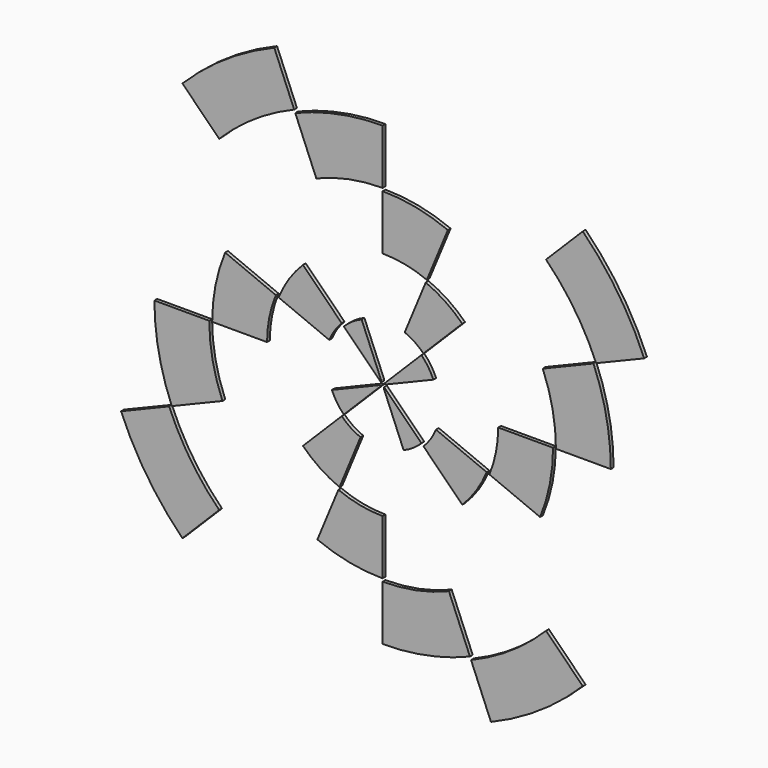
from build123d import *

# Parameters (mm, degrees)
F1_DEPTH = 1.2


# Not quite as in the source:
# - ends of sketch curves that miss each other by under 0.0002 mm in the source are joined


with BuildPart() as f1:
    # F0 (on Front) → F1 (new body)
    with BuildSketch(Plane.XZ):
        with BuildLine():
            Line((-1.2989994546, 0.0015044786), (15.0476048994, 6.7724896142))
            ThreePointArc((15.0476048994, 6.7724896142), (13.2918164287, 10.0573388369), (10.928922648, 12.9365332644))
            Line((10.928922648, 12.9365332644), (-2.0061062491, 0.0015044765))
            Line((-2.0061062498, 0.0015044786), (-1.2989994546, 0.0015044786))
        make_face()
    extrude(amount=F1_DEPTH)


with BuildPart() as f1b:
    # F0 (on Front) → F1, piece 2 (new body)
    with BuildSketch(Plane.XZ):
        with BuildLine():
            Line((11.6360294322, 13.6436400426), (25.0710583314, 27.0786688285))
            ThreePointArc((25.0710583314, 27.0786688285), (19.1611329685, 31.9288192702), (12.4185477522, 35.532806188))
            Line((12.4185477522, 35.532806188), (5.1475624685, 17.9790950988))
            ThreePointArc((5.1475624685, 17.9790950988), (8.6052984769, 16.1308966794), (11.6360294322, 13.6436400426))
        make_face()
    extrude(amount=F1_DEPTH)


with BuildPart() as f1c:
    # F0 (on Front) → F1, piece 3 (new body)
    with BuildSketch(Plane.XZ):
        with BuildLine():
            Line((12.8012311882, 36.4566857191), (20.0722164719, 54.0103968083))
            ThreePointArc((20.0722164719, 54.0103968083), (9.0042229134, 57.3678359894), (-2.5061061445, 58.5015044786))
            Line((-2.5061061445, 58.5015044786), (-2.5061062512, 39.5015044786))
            ThreePointArc((-2.5061062512, 39.5015044786), (5.2975067418, 38.7329156724), (12.8012311882, 36.4566857191))
        make_face()
    extrude(amount=F1_DEPTH)


with BuildPart() as f1d:
    # F0 (on Front) → F1, piece 4 (new body)
    with BuildSketch(Plane.XZ):
        with BuildLine():
            Line((-2.5061062512, 59.5015044786), (-2.5061062512, 78.5015044786))
            ThreePointArc((-2.5061062512, 78.5015044786), (-17.918241492, 76.9835416699), (-32.7380971661, 72.4879876471))
            Line((-32.7380971661, 72.4879876471), (-25.4671120094, 54.9342765053))
            ThreePointArc((-25.4671120094, 54.9342765053), (-14.2115254214, 58.3486213327), (-2.5061062512, 59.5015044786))
        make_face()
    extrude(amount=F1_DEPTH)


with BuildPart() as f1e:
    # F0 (on Front) → F1, piece 5 (new body)
    with BuildSketch(Plane.XZ):
        with BuildLine():
            ThreePointArc((-59.0746485757, 56.0700471439), (-46.9517246823, 66.0190736034), (-33.1207805954, 73.4118671809))
            Line((-33.1207805954, 73.4118671809), (-40.0090823229, 90.041698789))
            ThreePointArc((-40.0090823229, 90.041698789), (-56.9519888293, 80.9855266564), (-71.8025705987, 68.7979692436))
            Line((-71.8025705987, 68.7979692436), (-59.0746485757, 56.0700471439))
        make_face()
    extrude(amount=F1_DEPTH)


with BuildPart() as f1f:
    # F0 (on Front) → F1, piece 6 (new body)
    with BuildSketch(Plane.XZ):
        with BuildLine():
            Line((-15.9411350532, 12.9365333616), (-3.0061062497, 0.0015044801))
            Line((-3.0061062512, 0.0015044796), (-3.0061062512, 0.7086112711))
            Line((-3.0061062512, 0.7086112711), (-9.7770914079, 17.0552156204))
            ThreePointArc((-9.7770914079, 17.0552156204), (-13.0619406286, 15.2994271457), (-15.9411350532, 12.9365333616))
        make_face()
    extrude(amount=F1_DEPTH)


with BuildPart() as f1g:
    # F0 (on Front) → F1, piece 7 (new body)
    with BuildSketch(Plane.XZ):
        with BuildLine():
            Line((-16.6482418323, 13.6436401449), (-30.0832706344, 27.0786690279))
            ThreePointArc((-30.0832706344, 27.0786690279), (-34.933421069, 21.1687436591), (-38.5374079786, 14.4261584385))
            Line((-38.5374079786, 14.4261584385), (-20.9836968806, 7.155173176))
            ThreePointArc((-20.9836968806, 7.155173176), (-19.1354984654, 10.6129091865), (-16.6482418323, 13.6436401449))
        make_face()
    extrude(amount=F1_DEPTH)


with BuildPart() as f1h:
    # F0 (on Front) → F1, piece 8 (new body)
    with BuildSketch(Plane.XZ):
        with BuildLine():
            Line((-39.4612875101, 14.8088418734), (-57.0149986081, 22.0798271359))
            ThreePointArc((-57.0149986081, 22.0798271359), (-60.3724377655, 11.0118336257), (-61.5061062512, -0.4984953792))
            Line((-61.5061062512, -0.4984953792), (-42.5061062512, -0.498495425))
            ThreePointArc((-42.5061062512, -0.498495425), (-41.7375174473, 7.3051174597), (-39.4612875101, 14.8088418734))
        make_face()
    extrude(amount=F1_DEPTH)


with BuildPart() as f1i:
    # F0 (on Front) → F1, piece 9 (new body)
    with BuildSketch(Plane.XZ):
        with BuildLine():
            ThreePointArc((-81.5061062512, -0.498495331), (-79.9881434379, -15.9106307856), (-75.4925893833, -30.7304865244))
            Line((-75.4925893833, -30.7304865244), (-57.9388782503, -23.4595013464))
            ThreePointArc((-57.9388782503, -23.4595013464), (-61.3532231018, -12.2039147094), (-62.5061062512, -0.4984953768))
            Line((-62.5061062512, -0.4984953768), (-81.5061062512, -0.498495331))
        make_face()
    extrude(amount=F1_DEPTH)


with BuildPart() as f1j:
    # F0 (on Front) → F1, piece 10 (new body)
    with BuildSketch(Plane.XZ):
        with BuildLine():
            Line((-71.8025709327, -69.7949599525), (-59.0746488484, -57.0670379141))
            ThreePointArc((-59.0746488484, -57.0670379141), (-69.0236753224, -44.9441140327), (-76.4164689166, -31.1131699548))
            Line((-76.4164689166, -31.1131699548), (-93.0463005164, -38.0014717023))
            ThreePointArc((-93.0463005164, -38.0014717023), (-83.9901283634, -54.9443781978), (-71.8025709327, -69.7949599525))
        make_face()
    extrude(amount=F1_DEPTH)


with BuildPart() as f1k:
    # F0 (on Front) → F1, piece 11 (new body)
    with BuildSketch(Plane.XZ):
        with BuildLine():
            Line((-15.941135118, -13.9335243397), (-3.0061062521, -0.9984955205))
            Line((-3.0061062518, -0.9984955214), (-3.7132130396, -0.9984955214))
            Line((-3.7132130396, -0.9984955214), (-20.0598173842, -7.7694806994))
            ThreePointArc((-20.0598173842, -7.7694806994), (-18.3040289056, -11.0543299179), (-15.941135118, -13.9335243397))
        make_face()
    extrude(amount=F1_DEPTH)


with BuildPart() as f1l:
    # F0 (on Front) → F1, piece 12 (new body)
    with BuildSketch(Plane.XZ):
        with BuildLine():
            ThreePointArc((-30.0832707673, -28.0756599379), (-24.1733453927, -32.9258103653), (-17.4307601677, -36.5297972669))
            Line((-17.4307601677, -36.5297972669), (-10.1597749263, -18.9760861601))
            ThreePointArc((-10.1597749263, -18.9760861601), (-13.6175109391, -17.1278877491), (-16.6482419005, -14.6406311196))
            Line((-16.6482419005, -14.6406311196), (-30.0832707673, -28.0756599379))
        make_face()
    extrude(amount=F1_DEPTH)


with BuildPart() as f1m:
    # F0 (on Front) → F1, piece 13 (new body)
    with BuildSketch(Plane.XZ):
        with BuildLine():
            ThreePointArc((-25.0844288428, -55.0073879056), (-14.0164353111, -58.3648270531), (-2.5061062867, -59.4984955214))
            Line((-2.5061062512, -59.4984955214), (-2.5061062512, -40.4984955214))
            ThreePointArc((-2.5061062753, -40.4984955214), (-10.3097191732, -39.7299067293), (-17.8134436014, -37.4536767988))
            Line((-17.8134436014, -37.4536767988), (-25.0844288428, -55.0073879056))
        make_face()
    extrude(amount=F1_DEPTH)


with BuildPart() as f1n:
    # F0 (on Front) → F1, piece 14 (new body)
    with BuildSketch(Plane.XZ):
        with BuildLine():
            ThreePointArc((-2.5061062988, -79.4984955214), (12.9060291297, -77.9805326849), (27.7258848397, -73.4849786172))
            Line((27.7258848397, -73.4849786172), (20.4548996406, -55.9312674929))
            ThreePointArc((20.4548996406, -55.9312674929), (9.1993130255, -59.3456123544), (-2.5061062873, -60.4984955214))
            Line((-2.5061062512, -60.4984955214), (-2.5061062512, -79.4984955214))
        make_face()
    extrude(amount=F1_DEPTH)


with BuildPart() as f1o:
    # F0 (on Front) → F1, piece 15 (new body)
    with BuildSketch(Plane.XZ):
        with BuildLine():
            Line((66.7903582634, -69.7949601195), (54.0624362097, -57.0670380504))
            ThreePointArc((54.0624362097, -57.0670380504), (41.9395123403, -67.0160645391), (28.1085682712, -74.40885815))
            Line((28.1085682712, -74.40885815), (34.9968700388, -91.0386897414))
            ThreePointArc((34.9968700388, -91.0386897414), (51.9397765234, -81.9825175681), (66.7903582634, -69.7949601195))
        make_face()
    extrude(amount=F1_DEPTH)


with BuildPart() as f1p:
    # F0 (on Front) → F1, piece 16 (new body)
    with BuildSketch(Plane.XZ):
        with BuildLine():
            ThreePointArc((4.7648789479, -18.0522066457), (8.0497281643, -16.2964181631), (10.9289225833, -13.9335243721))
            Line((10.9289225833, -13.9335243721), (-2.0061062515, -0.9984955217))
            Line((-2.0061062512, -0.9984955216), (-2.0061062512, -1.7056023057))
            Line((-2.0061062512, -1.7056023057), (4.7648789479, -18.0522066457))
        make_face()
    extrude(amount=F1_DEPTH)


with BuildPart() as f1q:
    # F0 (on Front) → F1, piece 17 (new body)
    with BuildSketch(Plane.XZ):
        with BuildLine():
            ThreePointArc((25.0710581985, -28.0756600043), (29.9212086188, -22.1657346239), (33.5251955123, -15.4231493945))
            Line((33.5251955123, -15.4231493945), (15.9714843967, -8.1521641743))
            ThreePointArc((15.9714843967, -8.1521641743), (14.1232859899, -11.6099001893), (11.636029364, -14.6406311537))
            Line((11.636029364, -14.6406311537), (25.0710581985, -28.0756600043))
        make_face()
    extrude(amount=F1_DEPTH)


with BuildPart() as f1r:
    # F0 (on Front) → F1, piece 18 (new body)
    with BuildSketch(Plane.XZ):
        with BuildLine():
            ThreePointArc((52.0027861602, -23.0768180474), (55.3602252909, -12.0088245291), (56.4938937488, -0.4984955214))
            Line((56.4938937488, -0.4984955214), (37.4938937488, -0.4984955214))
            ThreePointArc((37.4938937488, -0.4984955214), (36.7253049638, -8.302108408), (34.4490750447, -15.8058328272))
            Line((34.4490750447, -15.8058328272), (52.0027861602, -23.0768180474))
        make_face()
    extrude(amount=F1_DEPTH)


with BuildPart() as f1s:
    # F0 (on Front) → F1, piece 19 (new body)
    with BuildSketch(Plane.XZ):
        with BuildLine():
            Line((57.4938937488, -0.4984955214), (76.4938937488, -0.4984955214))
            ThreePointArc((76.4938937488, -0.4984955214), (74.9759309355, 14.9136397428), (70.4803769538, 29.7334953056))
            Line((70.4803769538, 29.7334953056), (52.9266658033, 22.46251017))
            ThreePointArc((52.9266658033, 22.46251017), (56.3410105995, 11.2069236666), (57.4938937488, -0.4984955214))
        make_face()
    extrude(amount=F1_DEPTH)


with BuildPart() as f1t:
    # F0 (on Front) → F1, piece 20 (new body)
    with BuildSketch(Plane.XZ):
        with BuildLine():
            ThreePointArc((54.0624364823, 56.0700467349), (64.0114629272, 43.9471228295), (71.4042564881, 30.1161787338))
            Line((71.4042564881, 30.1161787338), (88.0340881044, 37.0044804412))
            ThreePointArc((88.0340881044, 37.0044804412), (78.9779159923, 53.9473869585), (66.7903585974, 68.7979687426))
            Line((66.7903585974, 68.7979687426), (54.0624364823, 56.0700467349))
        make_face()
    extrude(amount=F1_DEPTH)


solid = Compound([f1.part, f1b.part, f1c.part, f1d.part, f1e.part, f1f.part, f1g.part, f1h.part, f1i.part, f1j.part, f1k.part, f1l.part, f1m.part, f1n.part, f1o.part, f1p.part, f1q.part, f1r.part, f1s.part, f1t.part])
